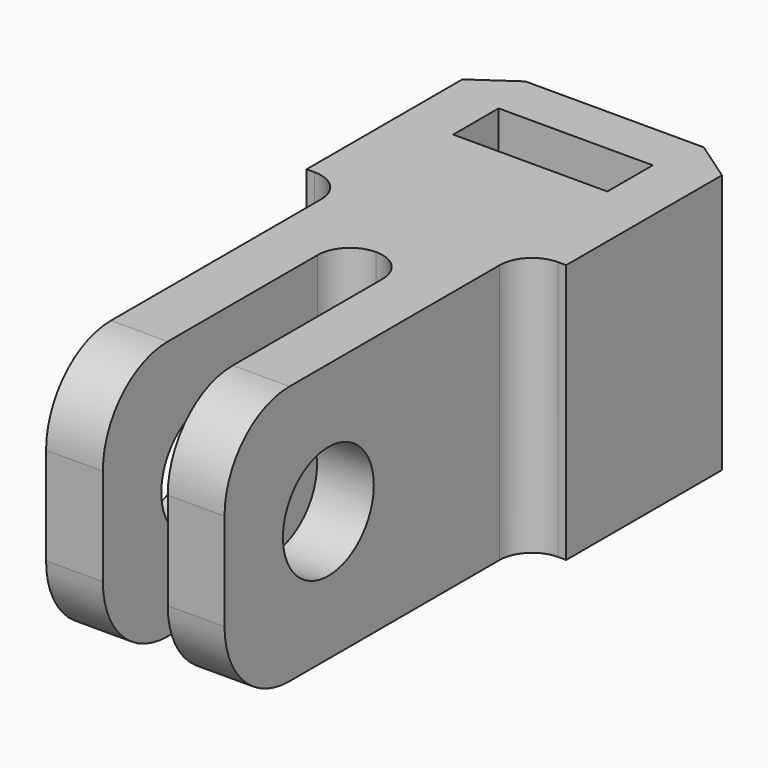
from build123d import *

# Parameters (mm, degrees)
F1_DEPTH = 16
F2_R     = 2.5
F3_DEPTH = 10
F4_R     = 3.5
F5_DEPTH = 11
F6_R     = 1.99999
F7_W     = 9.5
F7_H     = 3.5
F8_DEPTH = 12.3
F9_R     = 5


# Not quite as in the source:
# - a fillet or chamfer is up to 0.001 mm smaller than in the source, because OpenCascade refuses the exact size


with BuildPart() as f1:
    # F0 (on Top) → F1 (new body)
    with BuildSketch(Plane.XY):
        Polygon((-5.5, -2.8019716907), (-5.5, -26), (-2, -26), (-2, -7.4497503303), (2, -7.4497503303), (2, -26), (5.5, -26), (5.5, -2.8019716907), (8, -2.8019716907), (8, 9.1980283093), (5.5, 10.9290892892), (-5.5, 10.9290892892), (-8, 9.1980283093), (-8, -2.8019716907), align=None)
    extrude(amount=F1_DEPTH)

    # F2 (on face) → F3 (cut)
    with BuildSketch(Plane(origin=(0, 10.9290892892, 0), x_dir=(-1, 0, 0), z_dir=(0, 1, 0))):
        with Locations((0, 9)):
            Circle(F2_R)
    extrude(amount=-F3_DEPTH, mode=Mode.SUBTRACT)

    # F4 (on face) → F5 (cut, through all)
    with BuildSketch(Plane.YZ.offset(5.5)):
        with Locations((-18, 8)):
            Circle(F4_R)
    extrude(amount=-F5_DEPTH, mode=Mode.SUBTRACT)

    # F6 (radius 2 in the source; OpenCascade refuses exactly that, so slightly less here)
    f6_edges = [f1.edges().sort_by_distance(p)[0] for p in [
        (-5.5, -2.801972, 8),
        (2, -7.44975, 8),
        (-2, -7.44975, 8),
        (5.5, -2.801972, 8),
    ]]
    fillet(f6_edges, radius=F6_R)

    # F7 (on face) → F8 (cut)
    with BuildSketch(Plane.XY.offset(16)):
        with Locations((0, 6.1790892892)):
            Rectangle(F7_W, F7_H)
    extrude(amount=-F8_DEPTH, mode=Mode.SUBTRACT)

    # F9
    f9_edges = [f1.edges().sort_by_distance(p)[0] for p in [
        (3.75, -26, 16),
        (3.75, -26, 0),
        (-3.75, -26, 16),
        (-3.75, -26, 0),
    ]]
    fillet(f9_edges, radius=F9_R)


solid = f1.part
